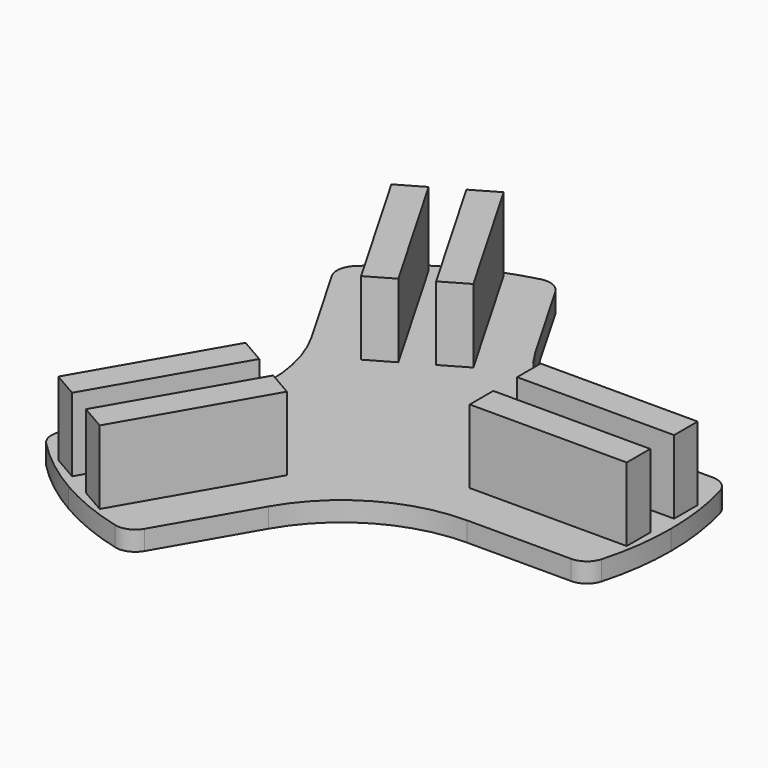
from build123d import *

# Parameters (mm, degrees)
F0_W           = 101.6
F0_H           = 19.05
F1_DEPTH       = 12.7
F2_DEPTH       = 9.525
F3_DEPTH       = 50.8
F4_D           = 4.7625
F4_DEPTH       = 12.7
F4_CSINK_D     = 11.0998
F4_CSINK_ANGLE = 90
F4_TIP         = 1.4307993491


with BuildPart() as f1:
    # F0 (on Top) → F1 (new body)
    with BuildSketch(Plane.XY):
        with BuildLine():
            Line((-88.9, -153.9793167929), (0, 0))
            Line((0, 0), (-88.9, 153.9793167929))
            ThreePointArc((-88.9, 153.9793167929), (-108.9975516555, 140.471967784), (-127.0733991266, 124.3591220394))
            ThreePointArc((-127.0733991266, 124.3591220394), (-130.596841253, 117.066025685), (-128.9952503885, 109.126327608))
            Line((-128.9952503885, 109.126327608), (-95.3205294432, 50.8))
            ThreePointArc((-95.3205294432, 50.8), (-81.7087104677, 0), (-95.3205294432, -50.8))
            Line((-95.3205294432, -50.8), (-128.9952503885, -109.126327608))
            ThreePointArc((-128.9952503885, -109.126327608), (-130.596841253, -117.066025685), (-127.0733991266, -124.3591220394))
            ThreePointArc((-127.0733991266, -124.3591220394), (-108.9975516555, -140.471967784), (-88.9, -153.9793167929))
        make_face()
        Polygon((-60.1282869611, -46.7410218803), (-43.630503019, -56.2660218803), (-94.430503019, -144.2542029048), (-110.9282869611, -134.7292029048), align=None, mode=Mode.SUBTRACT)
        Polygon((-43.630503019, 56.2660218803), (-60.1282869611, 46.7410218803), (-110.9282869611, 134.7292029048), (-94.430503019, 144.2542029048), align=None, mode=Mode.SUBTRACT)
        with BuildLine():
            Line((0, 0), (177.8, 0))
            ThreePointArc((177.8, 0), (176.1510684483, 24.1586647919), (171.2348584417, 47.8692307692))
            ThreePointArc((171.2348584417, 47.8692307692), (166.6805727898, 54.5671693366), (159.0037971245, 57.15))
            Line((159.0037971245, 57.15), (91.6543552339, 57.15))
            ThreePointArc((91.6543552339, 57.15), (40.8543552339, 70.7618189755), (3.6661742094, 107.95))
            Line((3.6661742094, 107.95), (-30.008546736, 166.276327608))
            ThreePointArc((-30.008546736, 166.276327608), (-36.0837315368, 171.6331950216), (-44.1614593151, 172.2283528086))
            ThreePointArc((-44.1614593151, 172.2283528086), (-67.1535167928, 164.630632576), (-88.9, 153.9793167929))
            Line((-88.9, 153.9793167929), (0, 0))
        make_face()
        Polygon((-10.4147688666, 75.4431349345), (-26.9125528087, 65.9181349345), (-77.7125528087, 153.906315959), (-61.2147688666, 163.431315959), align=None, mode=Mode.SUBTRACT)
        with Locations((121.3430558277, 19.1771130542)):
            Rectangle(F0_W, F0_H, mode=Mode.SUBTRACT)
        with BuildLine():
            ThreePointArc((159.0037971245, -57.15), (166.6805727898, -54.5671693366), (171.2348584417, -47.8692307692))
            ThreePointArc((171.2348584417, -47.8692307692), (176.1510684483, -24.1586647919), (177.8, 0))
            Line((177.8, 0), (0, 0))
            Line((0, 0), (-88.9, -153.9793167929))
            ThreePointArc((-88.9, -153.9793167929), (-67.1535167928, -164.630632576), (-44.1614593151, -172.2283528086))
            ThreePointArc((-44.1614593151, -172.2283528086), (-36.0837315368, -171.6331950216), (-30.008546736, -166.276327608))
            Line((-30.008546736, -166.276327608), (3.6661742094, -107.95))
            ThreePointArc((3.6661742094, -107.95), (40.8543552339, -70.7618189755), (91.6543552339, -57.15))
            Line((91.6543552339, -57.15), (159.0037971245, -57.15))
        make_face()
        Polygon((-26.9125528087, -65.9181349345), (-10.4147688666, -75.4431349345), (-61.2147688666, -163.431315959), (-77.7125528087, -153.906315959), align=None, mode=Mode.SUBTRACT)
        with Locations((121.3430558277, -19.1771130542)):
            Rectangle(F0_W, F0_H, mode=Mode.SUBTRACT)
    extrude(amount=F1_DEPTH)

    # F0 (on Top) → F2 (join)
    with BuildSketch(Plane.XY):
        Polygon((-94.430503019, -144.2542029048), (-43.630503019, -56.2660218803), (-60.1282869611, -46.7410218803), (-110.9282869611, -134.7292029048), align=None)
        Polygon((-61.2147688666, -163.431315959), (-10.4147688666, -75.4431349345), (-26.9125528087, -65.9181349345), (-77.7125528087, -153.906315959), align=None)
        with Locations((121.3430558277, -19.1771130542)):
            Rectangle(F0_W, F0_H)
        with Locations((121.3430558277, 19.1771130542)):
            Rectangle(F0_W, F0_H)
        Polygon((-77.7125528087, 153.906315959), (-26.9125528087, 65.9181349345), (-10.4147688666, 75.4431349345), (-61.2147688666, 163.431315959), align=None)
        Polygon((-110.9282869611, 134.7292029048), (-60.1282869611, 46.7410218803), (-43.630503019, 56.2660218803), (-94.430503019, 144.2542029048), align=None)
    extrude(amount=F2_DEPTH)

    # F3 (add): faces of the model
    f3_faces = [f1.faces().sort_by_distance(p)[0] for p in [
        (-77.2793949901, -95.4976123925, 9.525),
        (-44.0636608377, -114.6747254468, 9.525),
        (121.3430558277, -19.1771130542, 9.525),
        (121.3430558277, 19.1771130542, 9.525),
        (-44.0636608377, 114.6747254468, 9.525),
        (-77.2793949901, 95.4976123925, 9.525),
    ]]
    extrude(f3_faces, amount=F3_DEPTH)

    # F4
    with Locations(Plane(origin=(0, 0, 0), x_dir=(1, 0, 0), z_dir=(0, 0, -1))):
        with Locations((-93.1543949901, 122.9939189627), (-59.9386608377, 142.1710320169), (-28.1886608377, 87.1784188766), (-61.4043949901, 68.0013058224), (89.5930558277, 19.1771130542), (153.0930558277, 19.1771130542), (153.0930558277, -19.1771130542), (89.5930558277, -19.1771130542), (-61.4043949901, -68.0013058224), (-28.1886608377, -87.1784188766), (-59.9386608377, -142.1710320169), (-93.1543949901, -122.9939189627)):
            CounterSinkHole(F4_D / 2, F4_CSINK_D / 2, depth=F4_DEPTH, counter_sink_angle=F4_CSINK_ANGLE)
            with Locations((0, 0, -(F4_DEPTH + F4_TIP / 2))):  # 118° drill point
                Cone(0, F4_D / 2, F4_TIP, mode=Mode.SUBTRACT)


solid = f1.part
